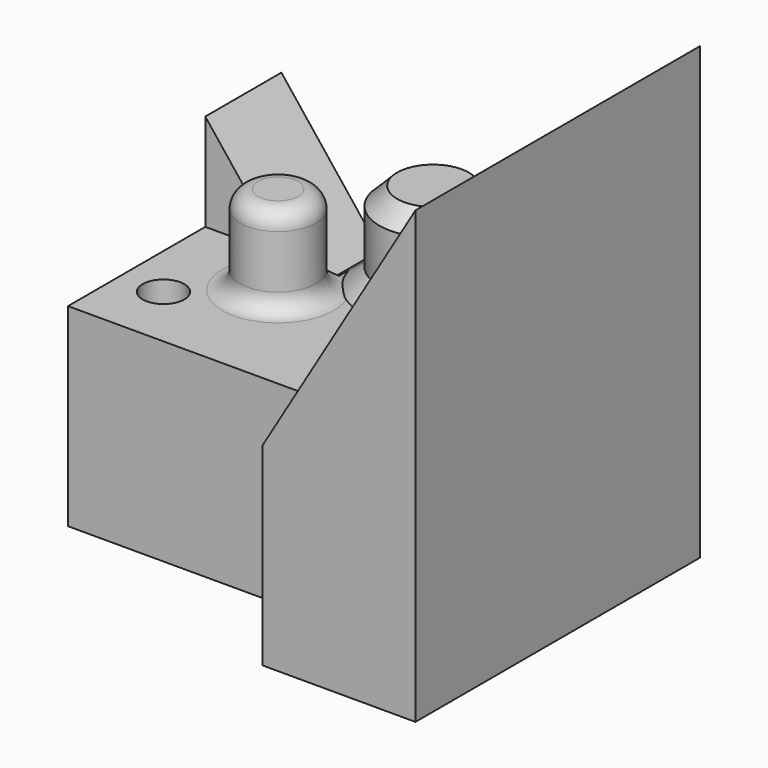
from build123d import *

# Parameters (mm, degrees)
F1_DEPTH = 76.2
F3_DEPTH = 25.4
F5_DEPTH = 49.022
F6_R     = 15.3034000689
F6_R_2   = 10.835787307
F6_R_3   = 5.9493654503
F7_DEPTH = 25.4
F8_DEPTH = 12.7
F9_DEPTH = 120.396


# Not quite as in the source:
# - a fillet or chamfer that OpenCascade refuses, or shapes differently, is made with other operations: its cross-section is extruded or revolved along the edge and cut away or added


with BuildPart() as f1:
    # F0 (on Front) → F1 (new body)
    with BuildSketch(Plane.XZ):
        Polygon((43.6695814133, 73.2915997505), (0, 0), (-37.7974100411, 0), (-75.9054422379, 48.224221915), (-75.9054422379, -55.3548447788), (43.6695814133, -55.3548447788), align=None)
    extrude(amount=F1_DEPTH)

    # F2 (on face) → F3 (join)
    with BuildSketch(Plane.XZ.offset(76.2)):
        Polygon((43.6695814133, 73.2915997505), (0, 0), (0, -55.3548447788), (43.6695814133, -55.3548447788), align=None)
    extrude(amount=F3_DEPTH)

    # F4 (on face) → F5 (cut)
    with BuildSketch(Plane.XZ.offset(76.2)):
        Polygon((-75.9054422379, 0), (-37.7974100411, 0), (-75.9054422379, 48.224221915), align=None)
    extrude(amount=-F5_DEPTH, mode=Mode.SUBTRACT)

    # F6 (on face) → F7 (join)
    with BuildSketch(Plane.XY):
        with Locations((-18.1702096015, -18.0441774428)):
            Circle(F6_R)
        with Locations((-44.1785492003, -40.8460125327)):
            Circle(F6_R_2)
        with Locations((-63.5862797499, -57.4966222048)):
            Circle(F6_R_3)
    extrude(amount=F7_DEPTH)

    # F8 (cut): a face of the model
    f8_faces = [f1.faces().sort_by_distance(p)[0] for p in [
        (-56.8514261395, -13.589, 24.1121109575),
    ]]
    extrude(f8_faces, amount=-F8_DEPTH, mode=Mode.SUBTRACT)

    # F9 (cut): a face of the model
    f9_faces = [f1.faces().sort_by_distance(p)[0] for p in [
        (-63.5862797499, -57.4966222048, 25.4),
    ]]
    extrude(f9_faces, amount=-F9_DEPTH, mode=Mode.SUBTRACT)

    # F10: fillet of radius 5.08 on 3 edges, made by hand

    # F10_s1 → F10_t2 (revolve, cut)
    with BuildSketch(Plane.XZ.offset(40.8460125327)):
        with BuildLine():
            ThreePointArc((-33.3427618933, 20.32), (-34.8306594448, 23.9121024484), (-38.4227618933, 25.4))
            Line((-38.4227618933, 25.4), (-33.3427618933, 25.4))
            Line((-33.3427618933, 25.4), (-33.3427618933, 20.32))
        make_face()
    revolve(axis=Axis((-44.1785492003, -40.8460125327, 25.4), (0, 0, 1)), mode=Mode.SUBTRACT)


with BuildPart() as f10_tool4:
    # F10_s5 → F10_t6 (revolve)
    with BuildSketch(Plane.XZ.offset(40.8460125327)):
        with BuildLine():
            ThreePointArc((-28.2627618933, 0), (-31.8548643417, 1.4878975516), (-33.3427618933, 5.08))
            Line((-33.3427618933, 5.08), (-33.3427618933, 0))
            Line((-33.3427618933, 0), (-28.2627618933, 0))
        make_face()
    revolve(axis=Axis((-44.1785492003, -40.8460125327, 0), (0, 0, 1)))

    split(bisect_by=Plane.XZ.offset(27.178), keep=Keep.TOP)


with BuildPart() as f1_1:
    add(f1.part)

    # F10_t3: union F10_tool4
    add(f10_tool4.part)


with BuildPart() as f10_tool9:
    # F10_s10 → F10_t11 (revolve)
    with BuildSketch(Plane.XZ.offset(40.8460125327)):
        with BuildLine():
            ThreePointArc((-28.2627618933, 0), (-31.8548643417, 1.4878975516), (-33.3427618933, 5.08))
            Line((-33.3427618933, 5.08), (-33.3427618933, 0))
            Line((-33.3427618933, 0), (-28.2627618933, 0))
        make_face()
    revolve(axis=Axis((-44.1785492003, -40.8460125327, 0), (0, 0, 1)))

    split(bisect_by=Plane(origin=(-14.5296914395, 0, 18.3867553359), x_dir=(0, 1, 0), z_dir=(0.6200078307, 0, -0.7845956218)), keep=Keep.TOP)


with BuildPart() as f1_2:
    add(f1_1.part)

    # F10_t8: union F10_tool9
    add(f10_tool9.part)

    # F11: chamfer of 5.08 on 3 edges, made by hand


with BuildPart() as f11_tool2:
    # F11_s3 → F11_t4 (revolve)
    with BuildSketch(Plane.XZ.offset(18.0441774428)):
        Polygon((2.2131904673, 0), (-2.8668095327, 5.08), (-2.8668095327, 0), align=None)
    revolve(axis=Axis((-18.1702096015, -18.0441774428, 0), (0, 0, 1)))

    split(bisect_by=Plane.XZ, keep=Keep.TOP)

    split(bisect_by=Plane(origin=(-14.5296914395, 0, 18.3867553359), x_dir=(0, 1, 0), z_dir=(0.6200078307, 0, -0.7845956218)), keep=Keep.TOP)


with BuildPart() as f1_3:
    add(f1_2.part)

    # F11_t1: union F11_tool2
    add(f11_tool2.part)

    # F11_s7 → F11_t8 (revolve, cut)
    with BuildSketch(Plane.XZ.offset(18.0441774428)):
        Polygon((-2.8668095327, 20.32), (-7.9468095327, 25.4), (-2.8668095327, 25.4), align=None)
    revolve(axis=Axis((-18.1702096015, -18.0441774428, 25.4), (0, 0, 1)), mode=Mode.SUBTRACT)


solid = f1_3.part
